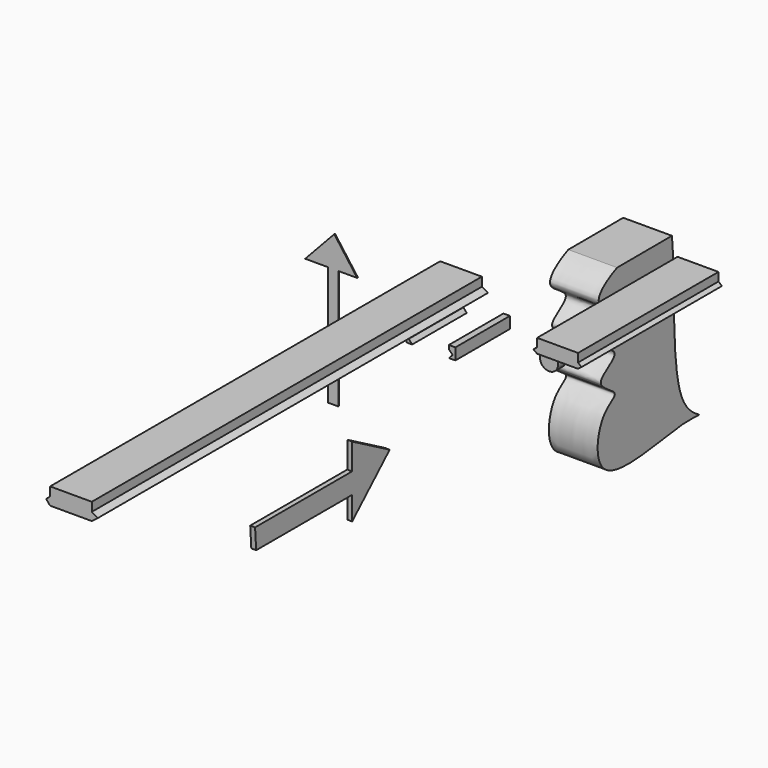
from build123d import *

# Parameters (mm, degrees)
F0_R      = 24.0061288108
F1_DEPTH  = 127
F2_W      = 11.2636005506
F2_H      = 2.7279288042
F3_DEPTH  = 23.495
F4_W      = 10.8573576435
F4_H      = 2.3079812527
F5_DEPTH  = 127
F7_DEPTH  = 12.7
F9_DEPTH  = 17.78
F10_R     = 2.3708686069
F11_DEPTH = 2.54
F13_DEPTH = 0.254
F15_DEPTH = 1.27
F17_DEPTH = 45.72


with BuildPart() as f1:
    # F0 (on Front) → F1 (new body)
    with BuildSketch(Plane.XZ):
        Circle(F0_R)
    extrude(amount=F1_DEPTH)

    # F2 (on Top) → F3 (join, symmetric)
    with BuildSketch(Plane.XY):
        with Locations((-0.0056633726, 1.3639644021)):
            Rectangle(F2_W, F2_H)
        Polygon((-6.6519216634, 3.6306970287), (-5.6374636479, 2.7279288042), (5.6261369027, 2.7279288042), (6.6812695004, 3.6359967198), (5.6261369027, 4.7706630105), (-5.6374636479, 4.7706630105), align=None)
    extrude(amount=F3_DEPTH, both=True)


with BuildPart() as f5:
    # F4 (on Front) → F5 (new body)
    with BuildSketch(Plane.XZ):
        with Locations((0, -25.2149105072)):
            Rectangle(F4_W, F4_H)
        Polygon((7.0078237914, -27.2799469531), (5.4286788218, -26.3689011335), (-5.4286788218, -26.3689011335), (-6.4756427892, -27.2799469531), (-5.4286788218, -28.4831065807), (5.4286788218, -28.4831065807), align=None)
    extrude(amount=F5_DEPTH)


with BuildPart() as f7:
    # F6 (on Right) → F7 (new body)
    with BuildSketch(Plane.YZ):
        with BuildLine():
            Line((52.7991135169, -33.7855707862), (34.947315381, -33.8373302608))
            add(Edge.make_bspline(
                [(34.947315381, -33.8373302608), (34.67488091, -33.9467110369), (31.757870512, -35.1920104732), (25.2745680521, -39.8272956488), (38.5548631415, -44.0824858907), (25.2312448829, -49.1199340969), (38.5238700761, -53.1982819393), (25.3841392291, -57.9482114221), (37.0845041004, -62.5762434591), (28.8690931811, -64.7132175953), (26.1553904819, -85.0723092199), (55.5084259962, -77.2703927863), (64.1606807814, -79.1247921103), (51.6549304079, -74.5162224387), (53.9403970758, -44.0065554038), (52.7991135169, -33.7855707862)],
                knots=[0.0617542874, 0.0617542874, 0.0617542874, 0.0617542874, 0.0681756693, 0.1295566744, 0.1894152283, 0.2473675483, 0.3038824598, 0.3618347798, 0.4183496913, 0.4675584285, 0.5485031035, 0.6638215709, 0.7141103583, 0.7802517263, 0.8977230327, 0.8977230327, 0.8977230327, 0.8977230327], degree=3))
        make_face()
    extrude(amount=F7_DEPTH)


with BuildPart() as f9:
    # F8 (on Front) → F9 (new body)
    with BuildSketch(Plane.XZ):
        Polygon((12.0650511235, -32.6633229852), (11.0542932525, -33.6740799248), (12.749758549, -33.6740799248), (12.749758549, -30.6744109839), (11.0542932525, -30.6744109839), (11.0542932525, -31.6525641829), align=None)
    extrude(amount=F9_DEPTH)


with BuildPart() as f9b:
    # F8 (on Front) → F9, piece 2 (new body)
    with BuildSketch(Plane.XZ):
        Polygon((0, -33.6740799248), (1.5010011848, -33.6740799248), (0.6206628168, -32.6633229852), (1.5010011848, -31.6525641829), (1.5010011848, -30.6744109839), (0, -30.6744109839), align=None)
    extrude(amount=F9_DEPTH)


with BuildPart() as f11:
    # F10 (on Front) → F11 (new body)
    with BuildSketch(Plane.XZ):
        with Locations((24.9688755721, -36.0097624362)):
            Circle(F10_R)
    extrude(amount=F11_DEPTH)


with BuildPart() as f13:
    # F12 (on Front) → F13 (new body)
    with BuildSketch(Plane.XZ):
        Polygon((-40.3839498758, -34.7523540258), (-34.475106746, -34.7523540258), (-34.475106746, -65.8208355308), (-31.7498035729, -65.8208355308), (-31.7498035729, -34.7523540258), (-26.8442537636, -34.7523540258), (-32.8178927302, -26.6516041011), align=None)
    extrude(amount=F13_DEPTH)


with BuildPart() as f15:
    # F14 (on Right) → F15 (new body)
    with BuildSketch(Plane.YZ):
        Polygon((-37.0261669159, -55.0077110529), (-68.6366707087, -55.0077110529), (-68.2774633169, -60.3958666325), (-37.0261669159, -60.3958666325), (-37.0261669159, -66.5024369955), (-24.8130224645, -55.0077110529), (-37.0261669159, -48.1827184558), align=None)
    extrude(amount=F15_DEPTH)


with BuildPart() as f17:
    # F16 (on Front) → F17 (new body)
    with BuildSketch(Plane.XZ):
        Polygon((67.0587420464, -5.1306844689), (67.0587420464, -2.9312425759), (56.3975758851, -2.9312425759), (56.3975758851, -5.1306844689), (55.4286055267, -5.8769658208), (56.3975758851, -6.5699419938), (67.0587420464, -6.5699419938), (67.9585010568, -5.8769658208), align=None)
    extrude(amount=F17_DEPTH)


solid = Compound([f5.part, f7.part, f9.part, f9b.part, f11.part, f13.part, f15.part, f17.part])
